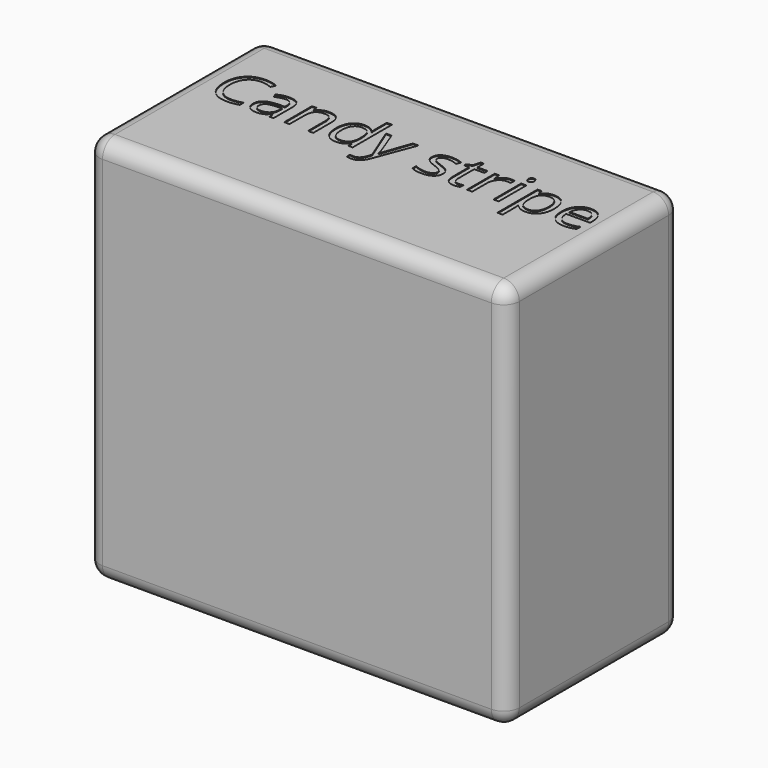
from build123d import *

# Parameters (mm, degrees)
F0_W         = 540
F0_H         = 280
F1_DEPTH     = 500
F2_R         = 20
F3_TEXT_SIZE = 83.3333333333
F4_DEPTH     = 1


# Not quite as in the source:
# - Text() gives the source's letters only with a copy of the font that has no kerning and outlines rounded to 1/6400 em; it was checked with that copy


with BuildPart() as f1:
    # F0 (on Top) → F1 (new body)
    with BuildSketch(Plane.XY):
        Rectangle(F0_W, F0_H)
    extrude(amount=F1_DEPTH)

    # F2
    f2_edges = [f1.edges().sort_by_distance(p)[0] for p in [
        (0, -140, 500),
        (270, 0, 500),
        (0, 140, 500),
        (-270, 0, 500),
        (270, 140, 250),
        (0, -140, 0),
        (270, 0, 0),
        (0, 140, 0),
        (-270, 0, 0),
        (-270, -140, 250),
        (270, -140, 250),
        (-270, 140, 250),
    ]]
    fillet(f2_edges, radius=F2_R)

    # F3 (on face) → F4 (cut)
    with BuildSketch(Plane.XY.offset(500)):
        with Locations((-240, 7.0395662842)):
            Text('Candy stripe', F3_TEXT_SIZE, font='Open Sans', text_align=(TextAlign.LEFT, TextAlign.BOTTOM))
    extrude(amount=-F4_DEPTH, mode=Mode.SUBTRACT)


solid = f1.part
